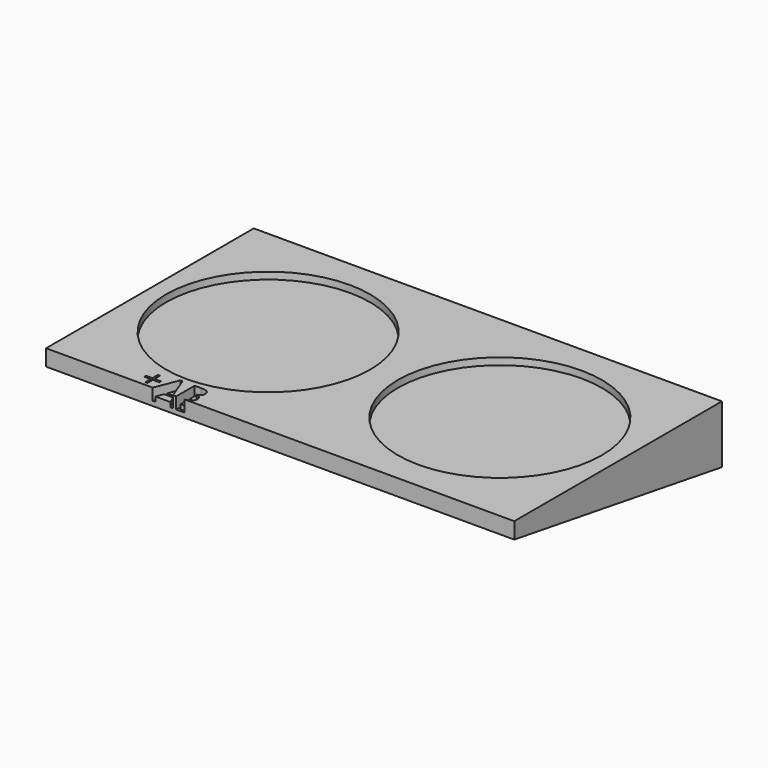
from build123d import *

# Parameters (mm, degrees)
F0_R          = 46
F0_R_2        = 44
F1_DEPTH      = 2
F0_TEXT_SIZE  = 13.8888888889
F2_DEPTH      = 2
F3_DEPTH      = 5
F6_DEPTH      = 101
F6_DEPTH_BACK = 101


# Not quite as in the source:
# - a feature of the source that left no trace in its solid (it failed there, or was rolled back) is left out
# - Text() gives the source's letters only with a copy of the font that has no kerning and outlines rounded to 1/6400 em; it was checked with that copy


with BuildPart() as f1:
    # F0 (on Top) → F1 (new body)
    with BuildSketch(Plane.XY):
        with BuildLine():
            Line((-41.3802083333, -56), (101, -56))
            Line((101, -56), (101, 56))
            Line((101, 56), (-101, 56))
            Line((-101, 56), (-101, -56))
            Line((-101, -56), (-54.9913194444, -56))
            Line((-54.9913194444, -56), (-51.0720486111, -46.0434027778))
            Line((-51.0720486111, -46.0434027778), (-50.1019965278, -46.0434027778))
            Line((-50.1019965278, -46.0434027778), (-46.2022569444, -56))
            Line((-46.2022569444, -56), (-44.8394097222, -56))
            Line((-44.8394097222, -56), (-44.8394097222, -46.0846354167))
            Line((-44.8394097222, -46.0846354167), (-42.0377604167, -46.0846354167))
            add(Edge.make_bspline(
                [(-42.0377604167, -46.0846354167), (-40.0651041667, -46.0846354167), (-39.1829427083, -46.6749131944)],
                knots=[0, 0, 0, 1, 1, 1], degree=2))
            add(Edge.make_bspline(
                [(-39.1829427083, -46.6749131944), (-38.30078125, -47.2651909722), (-38.30078125, -48.5390625)],
                knots=[0, 0, 0, 1, 1, 1], degree=2))
            add(Edge.make_bspline(
                [(-38.30078125, -48.5390625), (-38.30078125, -49.4223090278), (-38.7923177083, -49.9952256944)],
                knots=[0, 0, 0, 1, 1, 1], degree=2))
            add(Edge.make_bspline(
                [(-38.7923177083, -49.9952256944), (-39.2838541667, -50.5681423611), (-40.2278645833, -50.7374131944)],
                knots=[0, 0, 0, 1, 1, 1], degree=2))
            Line((-40.2278645833, -50.7374131944), (-40.2278645833, -50.8046875))
            add(Edge.make_bspline(
                [(-40.2278645833, -50.8046875), (-37.96875, -51.1909722222), (-37.96875, -53.1788194444)],
                knots=[0, 0, 0, 1, 1, 1], degree=2))
            add(Edge.make_bspline(
                [(-37.96875, -53.1788194444), (-37.96875, -54.5069444444), (-38.8671875, -55.2534722222)],
                knots=[0, 0, 0, 1, 1, 1], degree=2))
            add(Edge.make_bspline(
                [(-38.8671875, -55.2534722222), (-39.765625, -56), (-41.3802083333, -56)],
                knots=[0, 0, 0, 1, 1, 1], degree=2))
        make_face()
        Polygon((-58.5026041667, -47.7339409722), (-58.5026041667, -50.6354166667), (-55.7096354167, -50.6354166667), (-55.7096354167, -51.5707465278), (-58.5026041667, -51.5707465278), (-58.5026041667, -54.4613715278), (-59.4466145833, -54.4613715278), (-59.4466145833, -51.5707465278), (-62.2265625, -51.5707465278), (-62.2265625, -50.6354166667), (-59.4466145833, -50.6354166667), (-59.4466145833, -47.7339409722), align=None, mode=Mode.SUBTRACT)
        with Locations((-50, 0)):
            Circle(F0_R, mode=Mode.SUBTRACT)
        with Locations((50, 0)):
            Circle(F0_R, mode=Mode.SUBTRACT)
        with Locations((-50, 0)):
            Circle(F0_R)
        with Locations((-50, 0)):
            Circle(F0_R_2, mode=Mode.SUBTRACT)
        with Locations((50, 0)):
            Circle(F0_R)
        with Locations((50, 0)):
            Circle(F0_R_2, mode=Mode.SUBTRACT)
        with Locations((-50, 0)):
            Circle(F0_R_2)
        with Locations((50, 0)):
            Circle(F0_R_2)
    extrude(amount=F1_DEPTH)



with BuildPart() as f1b:
    # F0 (on Top) → F1, piece 2 (new body)
    with BuildSketch(Plane.XY):
        with BuildLine():
            Line((-52.1961805556, -51.8094618056), (-48.9887152778, -51.8094618056))
            Line((-48.9887152778, -51.8094618056), (-50.1432291667, -48.7365451389))
            add(Edge.make_bspline(
                [(-50.1432291667, -48.7365451389), (-50.3667534722, -48.1527777778), (-50.6032986111, -47.3064236111)],
                knots=[0, 0, 0, 1, 1, 1], degree=2))
            add(Edge.make_bspline(
                [(-50.6032986111, -47.3064236111), (-50.7530381944, -47.9574652778), (-51.0308159722, -48.7365451389)],
                knots=[0, 0, 0, 1, 1, 1], degree=2))
            Line((-51.0308159722, -48.7365451389), (-52.1961805556, -51.8094618056))
        make_face()
    extrude(amount=F1_DEPTH)


with BuildPart() as f1c:
    # F0 (on Top) → F1, piece 3 (new body)
    with BuildSketch(Plane.XY):
        Polygon((-53.8237847222, -56), (-47.3958333333, -56), (-48.6306423611, -52.8467881944), (-52.6041666667, -52.8467881944), align=None)
    extrude(amount=F1_DEPTH)


with BuildPart() as f1d:
    # F0 (on Top) → F1, piece 4 (new body)
    with BuildSketch(Plane.XY):
        with BuildLine():
            Line((-43.6870659722, -47.0828993056), (-43.6870659722, -50.3294270833))
            Line((-43.6870659722, -50.3294270833), (-41.7881944444, -50.3294270833))
            add(Edge.make_bspline(
                [(-41.7881944444, -50.3294270833), (-40.56640625, -50.3294270833), (-40.0303819444, -49.9463975694)],
                knots=[0, 0, 0, 1, 1, 1], degree=2))
            add(Edge.make_bspline(
                [(-40.0303819444, -49.9463975694), (-39.4943576389, -49.5633680556), (-39.4943576389, -48.65625)],
                knots=[0, 0, 0, 1, 1, 1], degree=2))
            add(Edge.make_bspline(
                [(-39.4943576389, -48.65625), (-39.4943576389, -47.8207465278), (-40.0911458333, -47.4518229167)],
                knots=[0, 0, 0, 1, 1, 1], degree=2))
            add(Edge.make_bspline(
                [(-40.0911458333, -47.4518229167), (-40.6879340278, -47.0828993056), (-41.9900173611, -47.0828993056)],
                knots=[0, 0, 0, 1, 1, 1], degree=2))
            Line((-41.9900173611, -47.0828993056), (-43.6870659722, -47.0828993056))
        make_face()
    extrude(amount=F1_DEPTH)


with BuildPart() as f1e:
    # F0 (on Top) → F1, piece 5 (new body)
    with BuildSketch(Plane.XY):
        with BuildLine():
            Line((-41.7122395833, -51.3059895833), (-43.6870659722, -51.3059895833))
            Line((-43.6870659722, -51.3059895833), (-43.6870659722, -55.0169270833))
            Line((-43.6870659722, -55.0169270833), (-41.6167534722, -55.0169270833))
            add(Edge.make_bspline(
                [(-41.6167534722, -55.0169270833), (-40.4166666667, -55.0169270833), (-39.8101128472, -54.5525173611)],
                knots=[0, 0, 0, 1, 1, 1], degree=2))
            add(Edge.make_bspline(
                [(-39.8101128472, -54.5525173611), (-39.2035590278, -54.0881076389), (-39.2035590278, -53.0963541667)],
                knots=[0, 0, 0, 1, 1, 1], degree=2))
            add(Edge.make_bspline(
                [(-39.2035590278, -53.0963541667), (-39.2035590278, -52.1740451389), (-39.82421875, -51.7400173611)],
                knots=[0, 0, 0, 1, 1, 1], degree=2))
            add(Edge.make_bspline(
                [(-39.82421875, -51.7400173611), (-40.4448784722, -51.3059895833), (-41.7122395833, -51.3059895833)],
                knots=[0, 0, 0, 1, 1, 1], degree=2))
        make_face()
    extrude(amount=F1_DEPTH)


with BuildPart() as f1_1:
    add(f1.part)

    add(f1b.part)  # F2 merges F1b

    add(f1c.part)  # F2 merges F1c

    add(f1d.part)  # F2 merges F1d

    add(f1e.part)  # F2 merges F1e
    # F1_face (on face) + F0 (on Top) → F2 (join)
    with BuildSketch(Plane(origin=(0.2527213924, 0.2779111323, 2), x_dir=(1, 0, 0), z_dir=(0, 0, 1))):
        with BuildLine():
            Line((-45.0921311146, -56.2779111323), (-45.0921311146, -46.3625465489))
            Line((-45.0921311146, -46.3625465489), (-42.290481809, -46.3625465489))
            add(Edge.make_bspline(
                [(-42.290481809, -46.3625465489), (-40.317825559, -46.3625465489), (-38.5535026424, -47.5431021045), (-38.5535026424, -49.7002201601), (-39.536575559, -50.8460534934), (-40.4805859757, -51.0153243267)],
                knots=[0, 0, 0, 1, 2, 2.6933560477, 3.3867120954, 3.3867120954, 3.3867120954], degree=2))
            Line((-40.4805859757, -51.0153243267), (-40.4805859757, -51.0825986323))
            add(Edge.make_bspline(
                [(-40.4805859757, -51.0825986323), (-38.2214713924, -51.4688833545), (-38.2214713924, -54.7848555767), (-40.0183463924, -56.2779111323), (-41.6329297257, -56.2779111323)],
                knots=[0, 0, 0, 1, 1.6681222707, 2.3362445415, 2.3362445415, 2.3362445415], degree=2))
            Line((-41.6329297257, -56.2779111323), (100.7472786076, -56.2779111323))
            Line((100.7472786076, -56.2779111323), (100.7472786076, 55.7220888677))
            Line((100.7472786076, 55.7220888677), (-101.2527213924, 55.7220888677))
            Line((-101.2527213924, 55.7220888677), (-101.2527213924, -56.2779111323))
            Line((-101.2527213924, -56.2779111323), (-55.2440408368, -56.2779111323))
            Line((-55.2440408368, -56.2779111323), (-51.3247700035, -46.3213139101))
            Line((-51.3247700035, -46.3213139101), (-50.3547179201, -46.3213139101))
            Line((-50.3547179201, -46.3213139101), (-46.4549783368, -56.2779111323))
            Line((-46.4549783368, -56.2779111323), (-45.0921311146, -56.2779111323))
        make_face()
        Polygon((-58.755325559, -48.0118521045), (-58.755325559, -50.9133277989), (-55.962356809, -50.9133277989), (-55.962356809, -51.8486576601), (-58.755325559, -51.8486576601), (-58.755325559, -54.7392826601), (-59.6993359757, -54.7392826601), (-59.6993359757, -51.8486576601), (-62.4792838924, -51.8486576601), (-62.4792838924, -50.9133277989), (-59.6993359757, -50.9133277989), (-59.6993359757, -48.0118521045), align=None, mode=Mode.SUBTRACT)
    with BuildSketch(Plane.XY):
        with BuildLine():
            Line((-41.3802083333, -56), (101, -56))
            Line((101, -56), (101, 56))
            Line((101, 56), (-101, 56))
            Line((-101, 56), (-101, -56))
            Line((-101, -56), (-54.9913194444, -56))
            Line((-54.9913194444, -56), (-51.0720486111, -46.0434027778))
            Line((-51.0720486111, -46.0434027778), (-50.1019965278, -46.0434027778))
            Line((-50.1019965278, -46.0434027778), (-46.2022569444, -56))
            Line((-46.2022569444, -56), (-44.8394097222, -56))
            Line((-44.8394097222, -56), (-44.8394097222, -46.0846354167))
            Line((-44.8394097222, -46.0846354167), (-42.0377604167, -46.0846354167))
            add(Edge.make_bspline(
                [(-42.0377604167, -46.0846354167), (-40.0651041667, -46.0846354167), (-39.1829427083, -46.6749131944)],
                knots=[0, 0, 0, 1, 1, 1], degree=2))
            add(Edge.make_bspline(
                [(-39.1829427083, -46.6749131944), (-38.30078125, -47.2651909722), (-38.30078125, -48.5390625)],
                knots=[0, 0, 0, 1, 1, 1], degree=2))
            add(Edge.make_bspline(
                [(-38.30078125, -48.5390625), (-38.30078125, -49.4223090278), (-38.7923177083, -49.9952256944)],
                knots=[0, 0, 0, 1, 1, 1], degree=2))
            add(Edge.make_bspline(
                [(-38.7923177083, -49.9952256944), (-39.2838541667, -50.5681423611), (-40.2278645833, -50.7374131944)],
                knots=[0, 0, 0, 1, 1, 1], degree=2))
            Line((-40.2278645833, -50.7374131944), (-40.2278645833, -50.8046875))
            add(Edge.make_bspline(
                [(-40.2278645833, -50.8046875), (-37.96875, -51.1909722222), (-37.96875, -53.1788194444)],
                knots=[0, 0, 0, 1, 1, 1], degree=2))
            add(Edge.make_bspline(
                [(-37.96875, -53.1788194444), (-37.96875, -54.5069444444), (-38.8671875, -55.2534722222)],
                knots=[0, 0, 0, 1, 1, 1], degree=2))
            add(Edge.make_bspline(
                [(-38.8671875, -55.2534722222), (-39.765625, -56), (-41.3802083333, -56)],
                knots=[0, 0, 0, 1, 1, 1], degree=2))
        make_face()
        Polygon((-58.5026041667, -47.7339409722), (-58.5026041667, -50.6354166667), (-55.7096354167, -50.6354166667), (-55.7096354167, -51.5707465278), (-58.5026041667, -51.5707465278), (-58.5026041667, -54.4613715278), (-59.4466145833, -54.4613715278), (-59.4466145833, -51.5707465278), (-62.2265625, -51.5707465278), (-62.2265625, -50.6354166667), (-59.4466145833, -50.6354166667), (-59.4466145833, -47.7339409722), align=None, mode=Mode.SUBTRACT)
        with Locations((-50, 0)):
            Circle(F0_R, mode=Mode.SUBTRACT)
        with Locations((50, 0)):
            Circle(F0_R, mode=Mode.SUBTRACT)
        Polygon((-53.8237847222, -56), (-47.3958333333, -56), (-48.6306423611, -52.8467881944), (-52.6041666667, -52.8467881944), align=None)
        with BuildLine():
            Line((-52.1961805556, -51.8094618056), (-48.9887152778, -51.8094618056))
            Line((-48.9887152778, -51.8094618056), (-50.1432291667, -48.7365451389))
            add(Edge.make_bspline(
                [(-50.1432291667, -48.7365451389), (-50.3667534722, -48.1527777778), (-50.6032986111, -47.3064236111)],
                knots=[0, 0, 0, 1, 1, 1], degree=2))
            add(Edge.make_bspline(
                [(-50.6032986111, -47.3064236111), (-50.7530381944, -47.9574652778), (-51.0308159722, -48.7365451389)],
                knots=[0, 0, 0, 1, 1, 1], degree=2))
            Line((-51.0308159722, -48.7365451389), (-52.1961805556, -51.8094618056))
        make_face()
        with BuildLine():
            Line((-43.6870659722, -47.0828993056), (-43.6870659722, -50.3294270833))
            Line((-43.6870659722, -50.3294270833), (-41.7881944444, -50.3294270833))
            add(Edge.make_bspline(
                [(-41.7881944444, -50.3294270833), (-40.56640625, -50.3294270833), (-40.0303819444, -49.9463975694)],
                knots=[0, 0, 0, 1, 1, 1], degree=2))
            add(Edge.make_bspline(
                [(-40.0303819444, -49.9463975694), (-39.4943576389, -49.5633680556), (-39.4943576389, -48.65625)],
                knots=[0, 0, 0, 1, 1, 1], degree=2))
            add(Edge.make_bspline(
                [(-39.4943576389, -48.65625), (-39.4943576389, -47.8207465278), (-40.0911458333, -47.4518229167)],
                knots=[0, 0, 0, 1, 1, 1], degree=2))
            add(Edge.make_bspline(
                [(-40.0911458333, -47.4518229167), (-40.6879340278, -47.0828993056), (-41.9900173611, -47.0828993056)],
                knots=[0, 0, 0, 1, 1, 1], degree=2))
            Line((-41.9900173611, -47.0828993056), (-43.6870659722, -47.0828993056))
        make_face()
        with BuildLine():
            Line((-41.7122395833, -51.3059895833), (-43.6870659722, -51.3059895833))
            Line((-43.6870659722, -51.3059895833), (-43.6870659722, -55.0169270833))
            Line((-43.6870659722, -55.0169270833), (-41.6167534722, -55.0169270833))
            add(Edge.make_bspline(
                [(-41.6167534722, -55.0169270833), (-40.4166666667, -55.0169270833), (-39.8101128472, -54.5525173611)],
                knots=[0, 0, 0, 1, 1, 1], degree=2))
            add(Edge.make_bspline(
                [(-39.8101128472, -54.5525173611), (-39.2035590278, -54.0881076389), (-39.2035590278, -53.0963541667)],
                knots=[0, 0, 0, 1, 1, 1], degree=2))
            add(Edge.make_bspline(
                [(-39.2035590278, -53.0963541667), (-39.2035590278, -52.1740451389), (-39.82421875, -51.7400173611)],
                knots=[0, 0, 0, 1, 1, 1], degree=2))
            add(Edge.make_bspline(
                [(-39.82421875, -51.7400173611), (-40.4448784722, -51.3059895833), (-41.7122395833, -51.3059895833)],
                knots=[0, 0, 0, 1, 1, 1], degree=2))
        make_face()
        with Locations((-62.9318576389, -56)):
            Text('+AB', F0_TEXT_SIZE, font='Open Sans', text_align=(TextAlign.LEFT, TextAlign.BOTTOM))
    extrude(amount=-F2_DEPTH)

    # F0 (on Top) → F3 (join)
    with BuildSketch(Plane.XY):
        with BuildLine():
            Line((-41.3802083333, -56), (101, -56))
            Line((101, -56), (101, 56))
            Line((101, 56), (-101, 56))
            Line((-101, 56), (-101, -56))
            Line((-101, -56), (-54.9913194444, -56))
            Line((-54.9913194444, -56), (-51.0720486111, -46.0434027778))
            Line((-51.0720486111, -46.0434027778), (-50.1019965278, -46.0434027778))
            Line((-50.1019965278, -46.0434027778), (-46.2022569444, -56))
            Line((-46.2022569444, -56), (-44.8394097222, -56))
            Line((-44.8394097222, -56), (-44.8394097222, -46.0846354167))
            Line((-44.8394097222, -46.0846354167), (-42.0377604167, -46.0846354167))
            add(Edge.make_bspline(
                [(-42.0377604167, -46.0846354167), (-40.0651041667, -46.0846354167), (-39.1829427083, -46.6749131944)],
                knots=[0, 0, 0, 1, 1, 1], degree=2))
            add(Edge.make_bspline(
                [(-39.1829427083, -46.6749131944), (-38.30078125, -47.2651909722), (-38.30078125, -48.5390625)],
                knots=[0, 0, 0, 1, 1, 1], degree=2))
            add(Edge.make_bspline(
                [(-38.30078125, -48.5390625), (-38.30078125, -49.4223090278), (-38.7923177083, -49.9952256944)],
                knots=[0, 0, 0, 1, 1, 1], degree=2))
            add(Edge.make_bspline(
                [(-38.7923177083, -49.9952256944), (-39.2838541667, -50.5681423611), (-40.2278645833, -50.7374131944)],
                knots=[0, 0, 0, 1, 1, 1], degree=2))
            Line((-40.2278645833, -50.7374131944), (-40.2278645833, -50.8046875))
            add(Edge.make_bspline(
                [(-40.2278645833, -50.8046875), (-37.96875, -51.1909722222), (-37.96875, -53.1788194444)],
                knots=[0, 0, 0, 1, 1, 1], degree=2))
            add(Edge.make_bspline(
                [(-37.96875, -53.1788194444), (-37.96875, -54.5069444444), (-38.8671875, -55.2534722222)],
                knots=[0, 0, 0, 1, 1, 1], degree=2))
            add(Edge.make_bspline(
                [(-38.8671875, -55.2534722222), (-39.765625, -56), (-41.3802083333, -56)],
                knots=[0, 0, 0, 1, 1, 1], degree=2))
        make_face()
        Polygon((-58.5026041667, -47.7339409722), (-58.5026041667, -50.6354166667), (-55.7096354167, -50.6354166667), (-55.7096354167, -51.5707465278), (-58.5026041667, -51.5707465278), (-58.5026041667, -54.4613715278), (-59.4466145833, -54.4613715278), (-59.4466145833, -51.5707465278), (-62.2265625, -51.5707465278), (-62.2265625, -50.6354166667), (-59.4466145833, -50.6354166667), (-59.4466145833, -47.7339409722), align=None, mode=Mode.SUBTRACT)
        with Locations((-50, 0)):
            Circle(F0_R, mode=Mode.SUBTRACT)
        with Locations((50, 0)):
            Circle(F0_R, mode=Mode.SUBTRACT)
        with Locations((-50, 0)):
            Circle(F0_R)
        with Locations((-50, 0)):
            Circle(F0_R_2, mode=Mode.SUBTRACT)
        with Locations((50, 0)):
            Circle(F0_R)
        with Locations((50, 0)):
            Circle(F0_R_2, mode=Mode.SUBTRACT)
    extrude(amount=F3_DEPTH)

    # F5 (on Right) → F6 (join, two sides)
    with BuildSketch(Plane.YZ) as f6_sk:
        Polygon((56, -20), (56, 0), (-56, 0), (-56, -2), align=None)
    extrude(amount=-F6_DEPTH)
    extrude(f6_sk.sketch, amount=F6_DEPTH_BACK)


solid = f1_1.part
